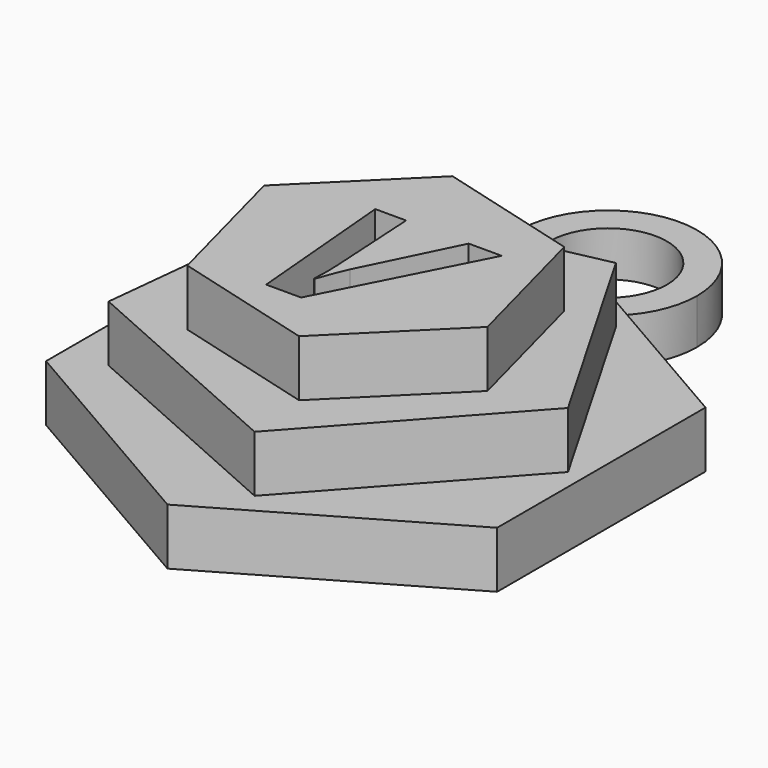
from build123d import *

# Parameters (mm, degrees)
F1_DEPTH     = 6.35
F3_DEPTH     = 6.35
F6_DEPTH     = 6.35
F7_TEXT_SIZE = 24.1305866641
F8_DEPTH     = 5.08
F10_DEPTH    = 5.08


# Not quite as in the source:
# - Text() gives the source's letters only with a copy of the font that has no kerning and outlines rounded to 1/6400 em; it was checked with that copy


with BuildPart() as f1:
    # F0 (on Top) → F1 (new body)
    with BuildSketch(Plane.XY):
        Polygon((25.4, -14.6646968374), (25.4, 14.6646968374), (0, 29.3293936748), (-25.4, 14.6646968374), (-25.4, -14.6646968374), (0, -29.3293936748), align=None)
    extrude(amount=F1_DEPTH)

    # F2 (on face) → F3 (join)
    with BuildSketch(Plane.XY.offset(6.35)):
        Polygon((23.6364481396, -2.4842908061), (9.6667651213, 21.7119099472), (-17.6620587334, 15.9029891142), (-20.5825177299, -11.8833221519), (4.9413632023, -23.2472861033), align=None)
    extrude(amount=F3_DEPTH)

    # F5 (on face) → F6 (join)
    with BuildSketch(Plane.XY.offset(12.7)):
        Polygon((4.2461514069, -16.1155809658), (16.0795782166, -4.3805154962), (11.8334268097, 11.7350654696), (-4.2461514069, 16.1155809658), (-16.0795782166, 4.3805154962), (-11.8334268097, -11.7350654696), align=None)
    extrude(amount=F6_DEPTH)

    # F7 (on face) → F8 (cut)
    with BuildSketch(Plane.XY.offset(19.05)):
        with Locations((-7.814422253, -10.248048231)):
            Text('V', F7_TEXT_SIZE, font='Open Sans', font_style=FontStyle.BOLDITALIC, text_align=(TextAlign.LEFT, TextAlign.BOTTOM))
    extrude(amount=-F8_DEPTH, mode=Mode.SUBTRACT)

    # F9 (on face) → F10 (join)
    with BuildSketch(Plane(origin=(0, 0, 0), x_dir=(1, 0, 0), z_dir=(0, 0, -1))):
        with BuildLine():
            ThreePointArc((-6.8326888559, -25.3845389246), (-3.9955376584, -41.9009563815), (10.0193779436, -32.7127240598))
            ThreePointArc((10.0193779436, -32.7127240598), (9.1882323217, -28.7171864014), (6.8326888559, -25.3845389246))
            Line((6.8326888559, -25.3845389246), (3.672741423, -27.2089354256))
            ThreePointArc((3.672741423, -27.2089354256), (5.8344728581, -29.5918835707), (6.6167, -32.7127240598))
            ThreePointArc((6.6167, -32.7127240598), (-3.1208404891, -38.5471969179), (-3.672741423, -27.2089354256))
            Line((-3.672741423, -27.2089354256), (-6.8326888559, -25.3845389246))
        make_face()
    extrude(amount=-F10_DEPTH)


solid = f1.part
